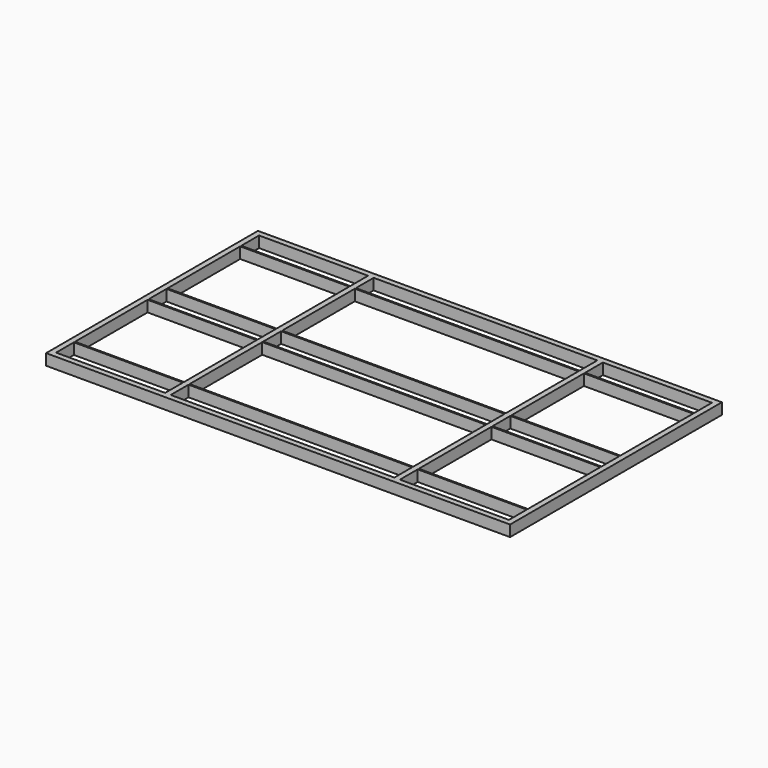
from build123d import *

# Parameters (mm, degrees)
F0_W     = 490
F0_H     = 6
F0_W_2   = 25
F1_DEPTH = 50


# Not quite as in the source:
# - a feature names something its author has since deleted; it is built from what else it names
# - the program builds the solid bodies; features that only make, move or delete a surface that nothing else refers to are left out


with BuildPart() as f1:
    # F0 (on Top) → F1 (new body)
    with BuildSketch(Plane.XY):
        Polygon((0, 1190), (0, 0), (515, 0), (540, 0), (540, 25), (540, 125), (540, 131), (540, 539), (540, 545), (540, 645), (540, 651), (540, 1059), (540, 1065), (540, 1165), (540, 1190), (515, 1190), align=None)
        Polygon((25, 1065), (25, 1165), (515, 1165), (515, 1065), (515, 1059), (515, 651), (515, 645), (515, 545), (515, 539), (515, 131), (515, 125), (515, 25), (25, 25), (25, 125), (25, 131), (25, 539), (25, 545), (25, 645), (25, 651), (25, 1059), align=None, mode=Mode.SUBTRACT)
        Polygon((540, 25), (540, 0), (1030, 0), (1055, 0), (1545, 0), (1570, 0), (1570, 25), (1570, 125), (1570, 131), (1570, 539), (1570, 545), (1570, 645), (1570, 651), (1570, 1059), (1570, 1065), (1570, 1165), (1570, 1190), (1545, 1190), (1055, 1190), (1030, 1190), (540, 1190), (540, 1165), (1030, 1165), (1055, 1165), (1545, 1165), (1545, 1065), (1545, 1059), (1545, 651), (1545, 645), (1545, 545), (1545, 539), (1545, 131), (1545, 125), (1545, 25), (1055, 25), (1030, 25), align=None)
        Polygon((1570, 25), (1570, 0), (2085, 0), (2085, 1190), (1570, 1190), (1570, 1165), (2060, 1165), (2060, 1065), (2060, 1059), (2060, 651), (2060, 645), (2060, 545), (2060, 539), (2060, 131), (2060, 125), (2060, 25), align=None)
        with Locations((270, 542)):
            Rectangle(F0_W, F0_H)
        with Locations((270, 128)):
            Rectangle(F0_W, F0_H)
        with Locations((270, 648)):
            Rectangle(F0_W, F0_H)
        with Locations((270, 1062)):
            Rectangle(F0_W, F0_H)
        with Locations((785, 648)):
            Rectangle(F0_W, F0_H)
        with Locations((1300, 648)):
            Rectangle(F0_W, F0_H)
        with Locations((1300, 542)):
            Rectangle(F0_W, F0_H)
        with Locations((785, 542)):
            Rectangle(F0_W, F0_H)
        with Locations((1815, 542)):
            Rectangle(F0_W, F0_H)
        with Locations((1815, 648)):
            Rectangle(F0_W, F0_H)
        with Locations((1815, 1062)):
            Rectangle(F0_W, F0_H)
        with Locations((1300, 1062)):
            Rectangle(F0_W, F0_H)
        with Locations((785, 1062)):
            Rectangle(F0_W, F0_H)
        with Locations((1815, 128)):
            Rectangle(F0_W, F0_H)
        with Locations((785, 128)):
            Rectangle(F0_W, F0_H)
        with Locations((1300, 128)):
            Rectangle(F0_W, F0_H)
        with Locations((1042.5, 128)):
            Rectangle(F0_W_2, F0_H)
        with Locations((1042.5, 542)):
            Rectangle(F0_W_2, F0_H)
        with Locations((1042.5, 1062)):
            Rectangle(F0_W_2, F0_H)
        with Locations((1042.5, 648)):
            Rectangle(F0_W_2, F0_H)
    extrude(amount=F1_DEPTH)


solid = f1.part
